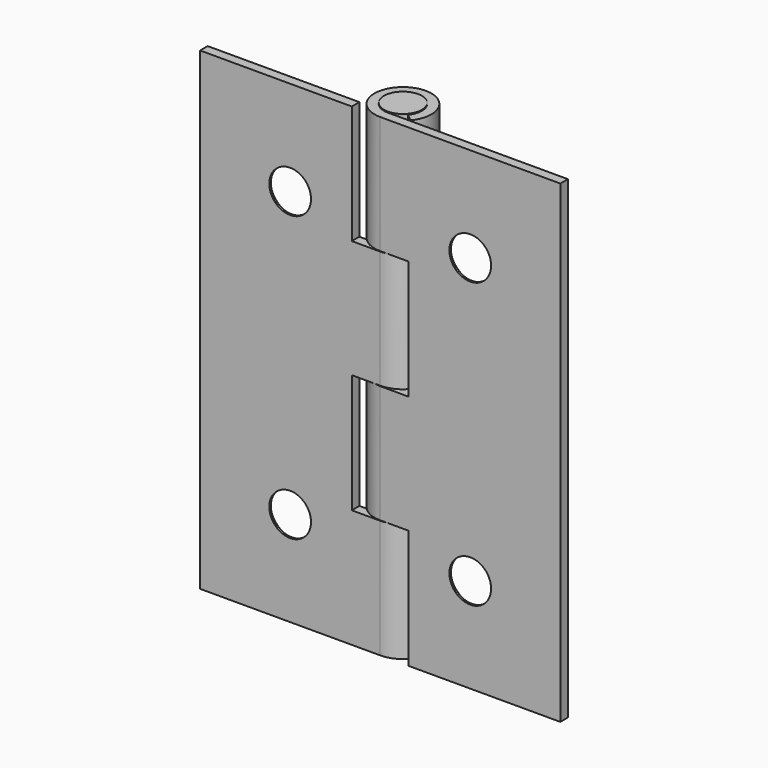
from build123d import *

# Parameters (mm, degrees)
F1_DEPTH          = 50
F3_DEPTH          = 50
F4_W              = 6
F4_H              = 0.05
F4_H_2            = 12.45
F4_H_3            = 12.5
F5_DEPTH          = 3.001
F5_DEPTH_BACK     = 3.001
F6_DEPTH          = 3.001
F6_DEPTH_BACK     = 3.001
F7_R              = 2
F8_DEPTH          = 50.1
F8_DEPTH_BACK     = 0.1
F10_D             = 4.4
F10_DEPTH         = 10
F10_CSINK_D       = 6
F10_CSINK_ANGLE   = 90
F10_TIP           = 1.3218933619
F10_2_D           = 4.4
F10_2_DEPTH       = 10
F10_2_CSINK_D     = 6
F10_2_CSINK_ANGLE = 90
F10_2_TIP         = 1.3218933619


with BuildPart() as f1:
    # F0 (on Top) → F1 (new body)
    with BuildSketch(Plane.XY):
        with BuildLine():
            Line((-19, -3), (0, -3))
            ThreePointArc((0, -3), (1.2247448714, -2.7386127875), (2.2360679775, -2))
            ThreePointArc((2.2360679775, -2), (0.0658067589, 2.9992781582), (-2.3216373532, -1.9))
            Line((-2.3216373532, -1.9), (-1.5477582355, -1.2666666667))
            ThreePointArc((-1.5477582355, -1.2666666667), (0.8563488386, 1.8073922282), (0, -2))
            Line((0, -2), (-19, -2))
            Line((-19, -2), (-19, -3))
        make_face()
    extrude(amount=-F1_DEPTH)

    # F4 (on Front) → F5 (cut, two sides)
    with BuildSketch(Plane.XZ) as f5_sk:
        with Locations((0, -37.475)):
            Rectangle(F4_W, F4_H)
        with Locations((0, -31.225)):
            Rectangle(F4_W, F4_H_2)
        with Locations((0, -24.975)):
            Rectangle(F4_W, F4_H)
        with Locations((0, -12.475)):
            Rectangle(F4_W, F4_H)
        with Locations((0, -6.2)):
            Rectangle(F4_W, F4_H_3)
    extrude(amount=-F5_DEPTH, mode=Mode.SUBTRACT)
    extrude(f5_sk.sketch, amount=F5_DEPTH_BACK, mode=Mode.SUBTRACT)

    # F10
    with Locations(Plane(origin=(0, -2, 0), x_dir=(-1, 0, 0), z_dir=(0, 1, 0))):
        with Locations((9.5, -10), (9.5, -40), (-9.5, -40), (-9.5, -10)):
            CounterSinkHole(F10_D / 2, F10_CSINK_D / 2, depth=F10_DEPTH, counter_sink_angle=F10_CSINK_ANGLE)
            with Locations((0, 0, -(F10_DEPTH + F10_TIP / 2))):  # 118° drill point
                Cone(0, F10_D / 2, F10_TIP, mode=Mode.SUBTRACT)


with BuildPart() as f3:
    # F2 (on Top) → F3 (new body)
    with BuildSketch(Plane.XY):
        with BuildLine():
            Line((1.5477582355, -1.2666666667), (2.3216373532, -1.9))
            ThreePointArc((2.3216373532, -1.9), (-1.2845232579, 2.7110883423), (0, -3))
            Line((0, -3), (19, -3))
            Line((19, -3), (19, -2))
            Line((19, -2), (0, -2))
            ThreePointArc((0, -2), (-0.8563488386, 1.8073922282), (1.5477582355, -1.2666666667))
        make_face()
    extrude(amount=-F3_DEPTH)

    # F4 (on Front) → F6 (cut, two sides)
    with BuildSketch(Plane.XZ) as f6_sk:
        with Locations((0, -43.75)):
            Rectangle(F4_W, F4_H_3)
        with Locations((0, -37.475)):
            Rectangle(F4_W, F4_H)
        with Locations((0, -24.975)):
            Rectangle(F4_W, F4_H)
        with Locations((0, -18.725)):
            Rectangle(F4_W, F4_H_2)
        with Locations((0, -12.475)):
            Rectangle(F4_W, F4_H)
    extrude(amount=-F6_DEPTH, mode=Mode.SUBTRACT)
    extrude(f6_sk.sketch, amount=F6_DEPTH_BACK, mode=Mode.SUBTRACT)

    # F10#2
    with Locations(Plane(origin=(0, -2, 0), x_dir=(-1, 0, 0), z_dir=(0, 1, 0))):
        with Locations((9.5, -10), (9.5, -40), (-9.5, -40), (-9.5, -10)):
            CounterSinkHole(F10_2_D / 2, F10_2_CSINK_D / 2, depth=F10_2_DEPTH, counter_sink_angle=F10_2_CSINK_ANGLE)
            with Locations((0, 0, -(F10_2_DEPTH + F10_2_TIP / 2))):  # 118° drill point
                Cone(0, F10_2_D / 2, F10_2_TIP, mode=Mode.SUBTRACT)


with BuildPart() as f8:
    # F7 (on Top) → F8 (new body, two sides)
    with BuildSketch(Plane.XY) as f8_sk:
        Circle(F7_R)
    extrude(amount=-F8_DEPTH)
    extrude(f8_sk.sketch, amount=F8_DEPTH_BACK)


solid = Compound([f1.part, f3.part, f8.part])
